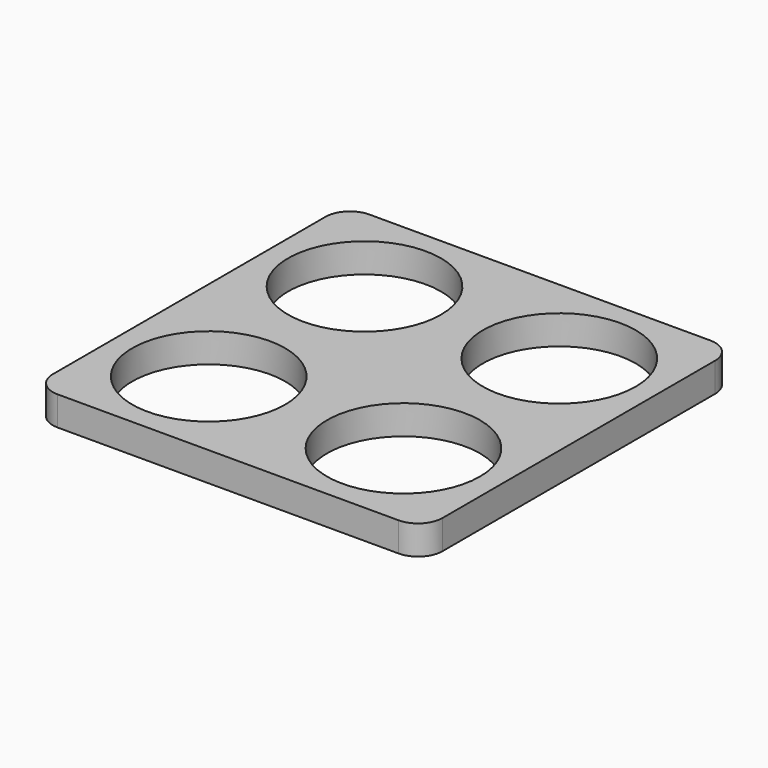
from build123d import *

# Parameters (mm, degrees)
F0_R     = 19.939
F1_DEPTH = 7.62


# Not quite as in the source:
# - a feature names something its author has since deleted; it is built from what else it names


with BuildPart() as f1:
    # F0 (on Top) → F1 (new body)
    with BuildSketch(Plane.XY):
        with BuildLine():
            ThreePointArc((-43.9448378141, -41.2645899475), (-42.0849658746, -45.754718008), (-37.5948378141, -47.6145899475))
            Line((-37.5948378141, -47.6145899475), (51.3051621859, -47.6145899475))
            ThreePointArc((51.3051621859, -47.6145899475), (55.7952902465, -45.754718008), (57.6551621859, -41.2645899475))
            Line((57.6551621859, -41.2645899475), (57.6551621859, 47.6354100525))
            ThreePointArc((57.6551621859, 47.6354100525), (55.7952902465, 52.1255381131), (51.3051621859, 53.9854100525))
            Line((51.3051621859, 53.9854100525), (-37.5948378141, 53.9854100525))
            ThreePointArc((-37.5948378141, 53.9854100525), (-42.0849658746, 52.1255381131), (-43.9448378141, 47.6354100525))
            Line((-43.9448378141, 47.6354100525), (-43.9448378141, -41.2645899475))
        make_face()
        with Locations((-18.5448378141, -22.2145899475)):
            Circle(F0_R, mode=Mode.SUBTRACT)
        with Locations((32.2551621859, -22.2145899475)):
            Circle(F0_R, mode=Mode.SUBTRACT)
        with Locations((-18.5448378141, 28.5854100525)):
            Circle(F0_R, mode=Mode.SUBTRACT)
        with Locations((32.2551621859, 28.5854100525)):
            Circle(F0_R, mode=Mode.SUBTRACT)
    extrude(amount=F1_DEPTH)


solid = f1.part
